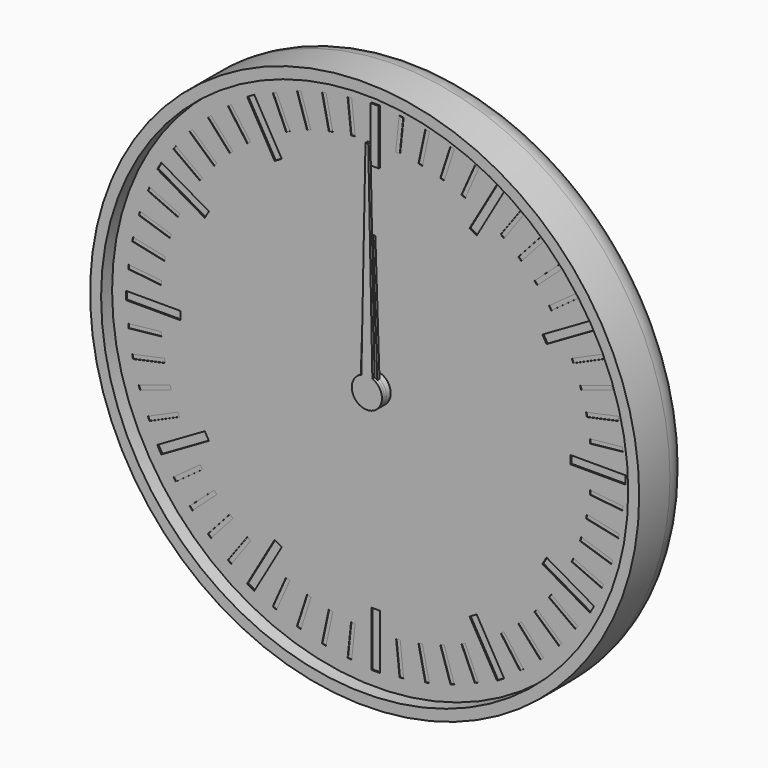
from build123d import *

# Parameters (mm, degrees)
F0_R      = 100
F1_DEPTH  = 24
F2_R      = 10
F3_T      = -4
F4_R      = 5.5
F4_R_2    = 3
F5_DEPTH  = 2
F6_DEPTH  = 19
F7_DEPTH  = 8
F9_DEPTH  = 4
F11_DEPTH = 4
F12_R     = 5.5
F12_R_2   = 3
F13_DEPTH = 2
F14_R     = 3
F15_DEPTH = 4
F17_DEPTH = 4
F18_R     = 3
F19_DEPTH = 2
F20_R     = 98
F20_R_2   = 5.5
F21_DEPTH = 1
F23_R     = 5
F23_R_2   = 3
F24_DEPTH = 2
F25_W     = 3
F25_H     = 20
F25_W_2   = 20
F25_H_2   = 3
F26_DEPTH = 0.5
F27_W     = 1.5
F27_H     = 12
F27_W_2   = 12
F27_H_2   = 1.5
F28_DEPTH = 0.2
F29_DEPTH = 1
F30_DEPTH = 0.4
F31_R     = 5.5
F31_R_2   = 3
F32_DEPTH = 5
F33_R     = 3
F34_DEPTH = 1
F36_DEPTH = 1


with BuildPart() as f1:
    # F0 (on Front) → F1 (new body)
    with BuildSketch(Plane.XZ):
        Circle(F0_R)
    extrude(amount=F1_DEPTH)

    # F2
    f2_edges = [f1.edges().sort_by_distance(p)[0] for p in [
        (-100, 0, 0),
    ]]
    fillet(f2_edges, radius=F2_R)

    # F3
    f3_openings = [f1.faces().sort_by_distance(p)[0] for p in [
        (0, -24, 0),
    ]]
    offset(amount=F3_T, openings=f3_openings)

    # F4 (on face) → F5 (join)
    with BuildSketch(Plane.XZ.offset(4)):
        Circle(F4_R)
        Circle(F4_R_2, mode=Mode.SUBTRACT)
        with Locations((40, 0)):
            Circle(F4_R)
        with Locations((40, 0)):
            Circle(F4_R_2, mode=Mode.SUBTRACT)
    extrude(amount=F5_DEPTH)


with BuildPart() as f6:
    # F6 (new): a face of the model
    f6_faces = [f1.part.faces().sort_by_distance(p)[0] for p in [
        (0, -4, 0),
    ]]
    extrude(f6_faces, amount=F6_DEPTH)

    # F8 (on face) → F9 (join)
    with BuildSketch(Plane.XZ.offset(6)):
        with BuildLine():
            ThreePointArc((9.2729637667, -1.3794085621), (9.3494561423, -0.6915886375), (9.375, 0))
            ThreePointArc((9.375, 0), (9.3494561423, 0.6915886375), (9.2729637667, 1.3794085621))
            ThreePointArc((9.2729637667, 1.3794085621), (8.9161548403, 2.8970343223), (8.3127812852, 4.3345463782))
            ThreePointArc((8.3127812852, 4.3345463782), (7.5845343223, 5.5104867402), (6.6911892658, 6.566476316))
            ThreePointArc((6.6911892658, 6.566476316), (5.5104867402, 7.5845343223), (4.1773988938, 8.3928519278))
            ThreePointArc((4.1773988938, 8.3928519278), (2.8970343223, 8.9161548403), (1.5536078905, 9.2453733036))
            ThreePointArc((1.5536078905, 9.2453733036), (0, 9.375), (-1.5536078905, 9.2453733036))
            ThreePointArc((-1.5536078905, 9.2453733036), (-2.8970343223, 8.9161548403), (-4.1773988938, 8.3928519278))
            ThreePointArc((-4.1773988938, 8.3928519278), (-5.5104867402, 7.5845343223), (-6.6911892658, 6.566476316))
            ThreePointArc((-6.6911892658, 6.566476316), (-7.5845343223, 5.5104867402), (-8.3127812852, 4.3345463782))
            ThreePointArc((-8.3127812852, 4.3345463782), (-8.9161548403, 2.8970343223), (-9.2729637667, 1.3794085621))
            ThreePointArc((-9.2729637667, 1.3794085621), (-9.375, 0), (-9.2729637667, -1.3794085621))
            ThreePointArc((-9.2729637667, -1.3794085621), (-8.9161548403, -2.8970343223), (-8.3127812852, -4.3345463782))
            ThreePointArc((-8.3127812852, -4.3345463782), (-7.5845343223, -5.5104867402), (-6.6911892658, -6.566476316))
            ThreePointArc((-6.6911892658, -6.566476316), (-5.5104867402, -7.5845343223), (-4.1773988938, -8.3928519278))
            ThreePointArc((-4.1773988938, -8.3928519278), (-2.8970343223, -8.9161548403), (-1.5536078905, -9.2453733036))
            ThreePointArc((-1.5536078905, -9.2453733036), (0, -9.375), (1.5536078905, -9.2453733036))
            ThreePointArc((1.5536078905, -9.2453733036), (2.8970343223, -8.9161548403), (4.1773988938, -8.3928519278))
            ThreePointArc((4.1773988938, -8.3928519278), (5.5104867402, -7.5845343223), (6.6911892658, -6.566476316))
            ThreePointArc((6.6911892658, -6.566476316), (7.5845343223, -5.5104867402), (8.3127812852, -4.3345463782))
            ThreePointArc((8.3127812852, -4.3345463782), (8.9161548403, -2.8970343223), (9.2729637667, -1.3794085621))
        make_face()
        with BuildLine():
            ThreePointArc((8.3127812852, 4.3345463782), (8.9161548403, 2.8970343223), (9.2729637667, 1.3794085621))
            Line((9.2729637667, 1.3794085621), (11.1823199426, 2.3946312492))
            Line((11.1823199426, 2.3946312492), (10.8182678729, 3.515068311))
            Line((10.8182678729, 3.515068311), (10.4542158031, 4.6355053728))
            Line((10.4542158031, 4.6355053728), (8.3127812852, 4.3345463782))
        make_face()
        with BuildLine():
            Line((11.1823199426, -2.3946312492), (9.2729637667, -1.3794085621))
            ThreePointArc((9.2729637667, -1.3794085621), (8.9161548403, -2.8970343223), (8.3127812852, -4.3345463782))
            Line((8.3127812852, -4.3345463782), (10.4542158031, -4.6355053728))
            Line((10.4542158031, -4.6355053728), (10.8182678729, -3.515068311))
            Line((10.8182678729, -3.515068311), (11.1823199426, -2.3946312492))
        make_face()
        with BuildLine():
            ThreePointArc((4.1773988938, 8.3928519278), (5.5104867402, 7.5845343223), (6.6911892658, 6.566476316))
            Line((6.6911892658, 6.566476316), (7.6391579371, 8.5101001246))
            Line((7.6391579371, 8.5101001246), (6.6860572448, 9.202568311))
            Line((6.6860572448, 9.202568311), (5.7329565525, 9.8950364974))
            Line((5.7329565525, 9.8950364974), (4.1773988938, 8.3928519278))
        make_face()
        with BuildLine():
            Line((7.6391579371, -8.5101001246), (6.6911892658, -6.566476316))
            ThreePointArc((6.6911892658, -6.566476316), (5.5104867402, -7.5845343223), (4.1773988938, -8.3928519278))
            Line((4.1773988938, -8.3928519278), (5.7329565525, -9.8950364974))
            Line((5.7329565525, -9.8950364974), (6.6860572448, -9.202568311))
            Line((6.6860572448, -9.202568311), (7.6391579371, -8.5101001246))
        make_face()
        with BuildLine():
            ThreePointArc((-1.5536078905, 9.2453733036), (0, 9.375), (1.5536078905, 9.2453733036))
            Line((1.5536078905, 9.2453733036), (1.1780972451, 11.375))
            Line((1.1780972451, 11.375), (0, 11.375))
            Line((0, 11.375), (-1.1780972451, 11.375))
            Line((-1.1780972451, 11.375), (-1.5536078905, 9.2453733036))
        make_face()
        with BuildLine():
            Line((1.1780972451, -11.375), (1.5536078905, -9.2453733036))
            ThreePointArc((1.5536078905, -9.2453733036), (0, -9.375), (-1.5536078905, -9.2453733036))
            Line((-1.5536078905, -9.2453733036), (-1.1780972451, -11.375))
            Line((-1.1780972451, -11.375), (0, -11.375))
            Line((0, -11.375), (1.1780972451, -11.375))
        make_face()
        with BuildLine():
            ThreePointArc((-6.6911892658, 6.566476316), (-5.5104867402, 7.5845343223), (-4.1773988938, 8.3928519278))
            Line((-4.1773988938, 8.3928519278), (-5.7329565525, 9.8950364974))
            Line((-5.7329565525, 9.8950364974), (-6.6860572448, 9.202568311))
            Line((-6.6860572448, 9.202568311), (-7.6391579371, 8.5101001246))
            Line((-7.6391579371, 8.5101001246), (-6.6911892658, 6.566476316))
        make_face()
        with BuildLine():
            Line((-5.7329565525, -9.8950364974), (-4.1773988938, -8.3928519278))
            ThreePointArc((-4.1773988938, -8.3928519278), (-5.5104867402, -7.5845343223), (-6.6911892658, -6.566476316))
            Line((-6.6911892658, -6.566476316), (-7.6391579371, -8.5101001246))
            Line((-7.6391579371, -8.5101001246), (-6.6860572448, -9.202568311))
            Line((-6.6860572448, -9.202568311), (-5.7329565525, -9.8950364974))
        make_face()
        with BuildLine():
            ThreePointArc((-9.2729637667, 1.3794085621), (-8.9161548403, 2.8970343223), (-8.3127812852, 4.3345463782))
            Line((-8.3127812852, 4.3345463782), (-10.4542158031, 4.6355053728))
            Line((-10.4542158031, 4.6355053728), (-10.8182678729, 3.515068311))
            Line((-10.8182678729, 3.515068311), (-11.1823199426, 2.3946312492))
            Line((-11.1823199426, 2.3946312492), (-9.2729637667, 1.3794085621))
        make_face()
        with BuildLine():
            Line((-10.4542158031, -4.6355053728), (-8.3127812852, -4.3345463782))
            ThreePointArc((-8.3127812852, -4.3345463782), (-8.9161548403, -2.8970343223), (-9.2729637667, -1.3794085621))
            Line((-9.2729637667, -1.3794085621), (-11.1823199426, -2.3946312492))
            Line((-11.1823199426, -2.3946312492), (-10.8182678729, -3.515068311))
            Line((-10.8182678729, -3.515068311), (-10.4542158031, -4.6355053728))
        make_face()
    extrude(amount=F9_DEPTH)

    # F35 (on face) → F36 (join)
    with BuildSketch(Plane.XZ.offset(23)):
        with BuildLine():
            ThreePointArc((-2, 5.123475383), (-3.1024184115, -4.5414755311), (5.5, 0))
            ThreePointArc((5.5, 0), (4.5414755311, 3.1024184115), (2, 5.123475383))
            ThreePointArc((2, 5.123475383), (0, 5.5), (-2, 5.123475383))
        make_face()
        with BuildLine():
            ThreePointArc((-2, 5.123475383), (0, 5.5), (2, 5.123475383))
            Line((2, 5.123475383), (0.5, 80))
            Line((0.5, 80), (0, 80))
            Line((0, 80), (-0.5, 80))
            Line((-0.5, 80), (-2, 5.123475383))
        make_face()
    extrude(amount=-F36_DEPTH)


with BuildPart() as f7:
    # F7 (new): a face of the model
    f7_faces = [f1.part.faces().sort_by_distance(p)[0] for p in [
        (40, -4, 0),
    ]]
    extrude(f7_faces, amount=F7_DEPTH)

    # F10 (on face) → F11 (join)
    with BuildSketch(Plane.XZ.offset(6)):
        with BuildLine():
            ThreePointArc((68.0829066802, -1.5381733945), (68.1144747006, -0.7693746225), (68.125, 0))
            ThreePointArc((68.125, 0), (68.1144747006, 0.7693746225), (68.0829066802, 1.5381733945))
            ThreePointArc((68.0829066802, 1.5381733945), (67.9709283072, 2.9398630294), (67.7890320221, 4.3342039956))
            ThreePointArc((67.7890320221, 4.3342039956), (67.5104012706, 5.8475163042), (67.1494235596, 7.3433252263))
            ThreePointArc((67.1494235596, 7.3433252263), (66.7484645208, 8.6911029668), (66.280643318, 10.0171558733))
            ThreePointArc((66.280643318, 10.0171558733), (65.6934659962, 11.4394680865), (65.0293803521, 12.8275385085))
            ThreePointArc((65.0293803521, 12.8275385085), (64.3569644814, 14.0625), (63.6236643925, 15.2623099717))
            ThreePointArc((63.6236643925, 15.2623099717), (62.7536029668, 16.5314602207), (61.815433119, 17.7511268046))
            ThreePointArc((61.815433119, 17.7511268046), (60.9009482166, 18.8192983038), (59.934217974, 19.8404278876))
            ThreePointArc((59.934217974, 19.8404278876), (58.8192983038, 20.9009482166), (57.6480467764, 21.8989056799))
            ThreePointArc((57.6480467764, 21.8989056799), (56.5314602207, 22.7536029668), (55.3735505752, 23.5514238999))
            ThreePointArc((55.3735505752, 23.5514238999), (54.0625, 24.3569644814), (52.709356105, 25.0895972944))
            ThreePointArc((52.709356105, 25.0895972944), (51.4394680865, 25.6934659962), (50.1409852457, 26.2331096755))
            ThreePointArc((50.1409852457, 26.2331096755), (48.6911029668, 26.7484645208), (47.2152055856, 27.1837531139))
            ThreePointArc((47.2152055856, 27.1837531139), (45.8475163042, 27.5104012706), (44.4652101991, 27.7682826779))
            ThreePointArc((44.4652101991, 27.7682826779), (42.9398630294, 27.9709283072), (41.4057159597, 28.0898484802))
            ThreePointArc((41.4057159597, 28.0898484802), (40, 28.125), (38.5942840403, 28.0898484802))
            ThreePointArc((38.5942840403, 28.0898484802), (37.0601369706, 27.9709283072), (35.5347898009, 27.7682826779))
            ThreePointArc((35.5347898009, 27.7682826779), (34.1524836958, 27.5104012706), (32.7847944144, 27.1837531139))
            ThreePointArc((32.7847944144, 27.1837531139), (31.3088970332, 26.7484645208), (29.8590147543, 26.2331096755))
            ThreePointArc((29.8590147543, 26.2331096755), (28.5605319135, 25.6934659962), (27.290643895, 25.0895972944))
            ThreePointArc((27.290643895, 25.0895972944), (25.9375, 24.3569644814), (24.6264494248, 23.5514238999))
            ThreePointArc((24.6264494248, 23.5514238999), (23.4685397793, 22.7536029668), (22.3519532236, 21.8989056799))
            ThreePointArc((22.3519532236, 21.8989056799), (21.1807016962, 20.9009482166), (20.065782026, 19.8404278876))
            ThreePointArc((20.065782026, 19.8404278876), (19.0990517834, 18.8192983038), (18.184566881, 17.7511268046))
            ThreePointArc((18.184566881, 17.7511268046), (17.2463970332, 16.5314602207), (16.3763356075, 15.2623099717))
            ThreePointArc((16.3763356075, 15.2623099717), (15.6430355186, 14.0625), (14.9706196479, 12.8275385085))
            ThreePointArc((14.9706196479, 12.8275385085), (14.3065340038, 11.4394680865), (13.719356682, 10.0171558733))
            ThreePointArc((13.719356682, 10.0171558733), (13.2515354792, 8.6911029668), (12.8505764404, 7.3433252263))
            ThreePointArc((12.8505764404, 7.3433252263), (12.4895987294, 5.8475163042), (12.2109679779, 4.3342039956))
            ThreePointArc((12.2109679779, 4.3342039956), (12.0290716928, 2.9398630294), (11.9170933198, 1.5381733945))
            ThreePointArc((11.9170933198, 1.5381733945), (11.875, 0), (11.9170933198, -1.5381733945))
            ThreePointArc((11.9170933198, -1.5381733945), (12.0290716928, -2.9398630294), (12.2109679779, -4.3342039956))
            ThreePointArc((12.2109679779, -4.3342039956), (12.4895987294, -5.8475163042), (12.8505764404, -7.3433252263))
            ThreePointArc((12.8505764404, -7.3433252263), (13.2515354792, -8.6911029668), (13.719356682, -10.0171558733))
            ThreePointArc((13.719356682, -10.0171558733), (14.3065340038, -11.4394680865), (14.9706196479, -12.8275385085))
            ThreePointArc((14.9706196479, -12.8275385085), (15.6430355186, -14.0625), (16.3763356075, -15.2623099717))
            ThreePointArc((16.3763356075, -15.2623099717), (17.2463970332, -16.5314602207), (18.184566881, -17.7511268046))
            ThreePointArc((18.184566881, -17.7511268046), (19.0990517834, -18.8192983038), (20.065782026, -19.8404278876))
            ThreePointArc((20.065782026, -19.8404278876), (21.1807016962, -20.9009482166), (22.3519532236, -21.8989056799))
            ThreePointArc((22.3519532236, -21.8989056799), (23.4685397793, -22.7536029668), (24.6264494248, -23.5514238999))
            ThreePointArc((24.6264494248, -23.5514238999), (25.9375, -24.3569644814), (27.290643895, -25.0895972944))
            ThreePointArc((27.290643895, -25.0895972944), (28.5605319135, -25.6934659962), (29.8590147543, -26.2331096755))
            ThreePointArc((29.8590147543, -26.2331096755), (31.3088970332, -26.7484645208), (32.7847944144, -27.1837531139))
            ThreePointArc((32.7847944144, -27.1837531139), (34.1524836958, -27.5104012706), (35.5347898009, -27.7682826779))
            ThreePointArc((35.5347898009, -27.7682826779), (37.0601369706, -27.9709283072), (38.5942840403, -28.0898484802))
            ThreePointArc((38.5942840403, -28.0898484802), (40, -28.125), (41.4057159597, -28.0898484802))
            ThreePointArc((41.4057159597, -28.0898484802), (42.9398630294, -27.9709283072), (44.4652101991, -27.7682826779))
            ThreePointArc((44.4652101991, -27.7682826779), (45.8475163042, -27.5104012706), (47.2152055856, -27.1837531139))
            ThreePointArc((47.2152055856, -27.1837531139), (48.6911029668, -26.7484645208), (50.1409852457, -26.2331096755))
            ThreePointArc((50.1409852457, -26.2331096755), (51.4394680865, -25.6934659962), (52.709356105, -25.0895972944))
            ThreePointArc((52.709356105, -25.0895972944), (54.0625, -24.3569644814), (55.3735505752, -23.5514238999))
            ThreePointArc((55.3735505752, -23.5514238999), (56.5314602207, -22.7536029668), (57.6480467764, -21.8989056799))
            ThreePointArc((57.6480467764, -21.8989056799), (58.8192983038, -20.9009482166), (59.934217974, -19.8404278876))
            ThreePointArc((59.934217974, -19.8404278876), (60.9009482166, -18.8192983038), (61.815433119, -17.7511268046))
            ThreePointArc((61.815433119, -17.7511268046), (62.7536029668, -16.5314602207), (63.6236643925, -15.2623099717))
            ThreePointArc((63.6236643925, -15.2623099717), (64.3569644814, -14.0625), (65.0293803521, -12.8275385085))
            ThreePointArc((65.0293803521, -12.8275385085), (65.6934659962, -11.4394680865), (66.280643318, -10.0171558733))
            ThreePointArc((66.280643318, -10.0171558733), (66.7484645208, -8.6911029668), (67.1494235596, -7.3433252263))
            ThreePointArc((67.1494235596, -7.3433252263), (67.5104012706, -5.8475163042), (67.7890320221, -4.3342039956))
            ThreePointArc((67.7890320221, -4.3342039956), (67.9709283072, -2.9398630294), (68.0829066802, -1.5381733945))
        make_face()
        with BuildLine():
            ThreePointArc((68.0829066802, 1.5381733945), (68.1144747006, 0.7693746225), (68.125, 0))
            ThreePointArc((68.125, 0), (68.1144747006, -0.7693746225), (68.0829066802, -1.5381733945))
            Line((68.0829066802, -1.5381733945), (70.125, -1.1780972451))
            Line((70.125, -1.1780972451), (70.125, 0))
            Line((70.125, 0), (70.125, 1.1780972451))
            Line((70.125, 1.1780972451), (68.0829066802, 1.5381733945))
        make_face()
        with BuildLine():
            ThreePointArc((67.1494235596, 7.3433252263), (67.5104012706, 5.8475163042), (67.7890320221, 4.3342039956))
            Line((67.7890320221, 4.3342039956), (69.7116366623, 5.1109866922))
            Line((69.7116366623, 5.1109866922), (69.4666964721, 6.2633396859))
            Line((69.4666964721, 6.2633396859), (69.2217562819, 7.4156926796))
            Line((69.2217562819, 7.4156926796), (67.1494235596, 7.3433252263))
        make_face()
        with BuildLine():
            Line((69.7116366623, -5.1109866922), (67.7890320221, -4.3342039956))
            ThreePointArc((67.7890320221, -4.3342039956), (67.5104012706, -5.8475163042), (67.1494235596, -7.3433252263))
            Line((67.1494235596, -7.3433252263), (69.2217562819, -7.4156926796))
            Line((69.2217562819, -7.4156926796), (69.4666964721, -6.2633396859))
            Line((69.4666964721, -6.2633396859), (69.7116366623, -5.1109866922))
        make_face()
        with BuildLine():
            ThreePointArc((65.0293803521, 12.8275385085), (65.6934659962, 11.4394680865), (66.280643318, 10.0171558733))
            Line((66.280643318, 10.0171558733), (67.9997322302, 11.1766959857))
            Line((67.9997322302, 11.1766959857), (67.5205569115, 12.2529413727))
            Line((67.5205569115, 12.2529413727), (67.0413815928, 13.3291867596))
            Line((67.0413815928, 13.3291867596), (65.0293803521, 12.8275385085))
        make_face()
        with BuildLine():
            Line((67.9997322302, -11.1766959857), (66.280643318, -10.0171558733))
            ThreePointArc((66.280643318, -10.0171558733), (65.6934659962, -11.4394680865), (65.0293803521, -12.8275385085))
            Line((65.0293803521, -12.8275385085), (67.0413815928, -13.3291867596))
            Line((67.0413815928, -13.3291867596), (67.5205569115, -12.2529413727))
            Line((67.5205569115, -12.2529413727), (67.9997322302, -11.1766959857))
        make_face()
        with BuildLine():
            ThreePointArc((61.815433119, 17.7511268046), (62.7536029668, 16.5314602207), (63.6236643925, 15.2623099717))
            Line((63.6236643925, 15.2623099717), (65.064105142, 16.753930033))
            Line((65.064105142, 16.753930033), (64.3716369555, 17.7070307253))
            Line((64.3716369555, 17.7070307253), (63.6791687691, 18.6601314176))
            Line((63.6791687691, 18.6601314176), (61.815433119, 17.7511268046))
        make_face()
        with BuildLine():
            Line((65.064105142, -16.753930033), (63.6236643925, -15.2623099717))
            ThreePointArc((63.6236643925, -15.2623099717), (62.7536029668, -16.5314602207), (61.815433119, -17.7511268046))
            Line((61.815433119, -17.7511268046), (63.6791687691, -18.6601314176))
            Line((63.6791687691, -18.6601314176), (64.3716369555, -17.7070307253))
            Line((64.3716369555, -17.7070307253), (65.064105142, -16.753930033))
        make_face()
        with BuildLine():
            ThreePointArc((57.6480467764, 21.8989056799), (58.8192983038, 20.9009482166), (59.934217974, 19.8404278876))
            Line((59.934217974, 19.8404278876), (61.0330563882, 21.5989369435))
            Line((61.0330563882, 21.5989369435), (60.1575595166, 22.3872378675))
            Line((60.1575595166, 22.3872378675), (59.282062645, 23.1755387915))
            Line((59.282062645, 23.1755387915), (57.6480467764, 21.8989056799))
        make_face()
        with BuildLine():
            Line((61.0330563882, -21.5989369435), (59.934217974, -19.8404278876))
            ThreePointArc((59.934217974, -19.8404278876), (58.8192983038, -20.9009482166), (57.6480467764, -21.8989056799))
            Line((57.6480467764, -21.8989056799), (59.282062645, -23.1755387915))
            Line((59.282062645, -23.1755387915), (60.1575595166, -22.3872378675))
            Line((60.1575595166, -22.3872378675), (61.0330563882, -21.5989369435))
        make_face()
        with BuildLine():
            ThreePointArc((52.709356105, 25.0895972944), (54.0625, 24.3569644814), (55.3735505752, 23.5514238999))
            Line((55.3735505752, 23.5514238999), (56.0827621424, 25.4999666665))
            Line((56.0827621424, 25.4999666665), (55.0625, 26.089015289))
            Line((55.0625, 26.089015289), (54.0422378576, 26.6780639116))
            Line((54.0422378576, 26.6780639116), (52.709356105, 25.0895972944))
        make_face()
        with BuildLine():
            Line((56.0827621424, -25.4999666665), (55.3735505752, -23.5514238999))
            ThreePointArc((55.3735505752, -23.5514238999), (54.0625, -24.3569644814), (52.709356105, -25.0895972944))
            Line((52.709356105, -25.0895972944), (54.0422378576, -26.6780639116))
            Line((54.0422378576, -26.6780639116), (55.0625, -26.089015289))
            Line((55.0625, -26.089015289), (56.0827621424, -25.4999666665))
        make_face()
        with BuildLine():
            ThreePointArc((47.2152055856, 27.1837531139), (48.6911029668, 26.7484645208), (50.1409852457, 26.2331096755))
            Line((50.1409852457, 26.2331096755), (50.4295740173, 28.2865254836))
            Line((50.4295740173, 28.2865254836), (49.3091369555, 28.6505775534))
            Line((49.3091369555, 28.6505775534), (48.1886998938, 29.0146296232))
            Line((48.1886998938, 29.0146296232), (47.2152055856, 27.1837531139))
        make_face()
        with BuildLine():
            Line((50.4295740173, -28.2865254836), (50.1409852457, -26.2331096755))
            ThreePointArc((50.1409852457, -26.2331096755), (48.6911029668, -26.7484645208), (47.2152055856, -27.1837531139))
            Line((47.2152055856, -27.1837531139), (48.1886998938, -29.0146296232))
            Line((48.1886998938, -29.0146296232), (49.3091369555, -28.6505775534))
            Line((49.3091369555, -28.6505775534), (50.4295740173, -28.2865254836))
        make_face()
        with BuildLine():
            ThreePointArc((41.4057159597, 28.0898484802), (42.9398630294, 27.9709283072), (44.4652101991, 27.7682826779))
            Line((44.4652101991, 27.7682826779), (44.3205634611, 29.8368274034))
            Line((44.3205634611, 29.8368274034), (43.1489199559, 29.959972098))
            Line((43.1489199559, 29.959972098), (41.9772764508, 30.0831167926))
            Line((41.9772764508, 30.0831167926), (41.4057159597, 28.0898484802))
        make_face()
        with BuildLine():
            Line((44.3205634611, -29.8368274034), (44.4652101991, -27.7682826779))
            ThreePointArc((44.4652101991, -27.7682826779), (42.9398630294, -27.9709283072), (41.4057159597, -28.0898484802))
            Line((41.4057159597, -28.0898484802), (41.9772764508, -30.0831167926))
            Line((41.9772764508, -30.0831167926), (43.1489199559, -29.959972098))
            Line((43.1489199559, -29.959972098), (44.3205634611, -29.8368274034))
        make_face()
        with BuildLine():
            ThreePointArc((35.5347898009, 27.7682826779), (37.0601369706, 27.9709283072), (38.5942840403, 28.0898484802))
            Line((38.5942840403, 28.0898484802), (38.0227235492, 30.0831167926))
            Line((38.0227235492, 30.0831167926), (36.8510800441, 29.959972098))
            Line((36.8510800441, 29.959972098), (35.6794365389, 29.8368274034))
            Line((35.6794365389, 29.8368274034), (35.5347898009, 27.7682826779))
        make_face()
        with BuildLine():
            Line((38.0227235492, -30.0831167926), (38.5942840403, -28.0898484802))
            ThreePointArc((38.5942840403, -28.0898484802), (37.0601369706, -27.9709283072), (35.5347898009, -27.7682826779))
            Line((35.5347898009, -27.7682826779), (35.6794365389, -29.8368274034))
            Line((35.6794365389, -29.8368274034), (36.8510800441, -29.959972098))
            Line((36.8510800441, -29.959972098), (38.0227235492, -30.0831167926))
        make_face()
        with BuildLine():
            ThreePointArc((29.8590147543, 26.2331096755), (31.3088970332, 26.7484645208), (32.7847944144, 27.1837531139))
            Line((32.7847944144, 27.1837531139), (31.8113001062, 29.0146296232))
            Line((31.8113001062, 29.0146296232), (30.6908630445, 28.6505775534))
            Line((30.6908630445, 28.6505775534), (29.5704259827, 28.2865254836))
            Line((29.5704259827, 28.2865254836), (29.8590147543, 26.2331096755))
        make_face()
        with BuildLine():
            Line((31.8113001062, -29.0146296232), (32.7847944144, -27.1837531139))
            ThreePointArc((32.7847944144, -27.1837531139), (31.3088970332, -26.7484645208), (29.8590147543, -26.2331096755))
            Line((29.8590147543, -26.2331096755), (29.5704259827, -28.2865254836))
            Line((29.5704259827, -28.2865254836), (30.6908630445, -28.6505775534))
            Line((30.6908630445, -28.6505775534), (31.8113001062, -29.0146296232))
        make_face()
        with BuildLine():
            ThreePointArc((24.6264494248, 23.5514238999), (25.9375, 24.3569644814), (27.290643895, 25.0895972944))
            Line((27.290643895, 25.0895972944), (25.9577621424, 26.6780639116))
            Line((25.9577621424, 26.6780639116), (24.9375, 26.089015289))
            Line((24.9375, 26.089015289), (23.9172378576, 25.4999666665))
            Line((23.9172378576, 25.4999666665), (24.6264494248, 23.5514238999))
        make_face()
        with BuildLine():
            Line((25.9577621424, -26.6780639116), (27.290643895, -25.0895972944))
            ThreePointArc((27.290643895, -25.0895972944), (25.9375, -24.3569644814), (24.6264494248, -23.5514238999))
            Line((24.6264494248, -23.5514238999), (23.9172378576, -25.4999666665))
            Line((23.9172378576, -25.4999666665), (24.9375, -26.089015289))
            Line((24.9375, -26.089015289), (25.9577621424, -26.6780639116))
        make_face()
        with BuildLine():
            ThreePointArc((20.065782026, 19.8404278876), (21.1807016962, 20.9009482166), (22.3519532236, 21.8989056799))
            Line((22.3519532236, 21.8989056799), (20.717937355, 23.1755387915))
            Line((20.717937355, 23.1755387915), (19.8424404834, 22.3872378675))
            Line((19.8424404834, 22.3872378675), (18.9669436118, 21.5989369435))
            Line((18.9669436118, 21.5989369435), (20.065782026, 19.8404278876))
        make_face()
        with BuildLine():
            Line((20.717937355, -23.1755387915), (22.3519532236, -21.8989056799))
            ThreePointArc((22.3519532236, -21.8989056799), (21.1807016962, -20.9009482166), (20.065782026, -19.8404278876))
            Line((20.065782026, -19.8404278876), (18.9669436118, -21.5989369435))
            Line((18.9669436118, -21.5989369435), (19.8424404834, -22.3872378675))
            Line((19.8424404834, -22.3872378675), (20.717937355, -23.1755387915))
        make_face()
        with BuildLine():
            ThreePointArc((16.3763356075, 15.2623099717), (17.2463970332, 16.5314602207), (18.184566881, 17.7511268046))
            Line((18.184566881, 17.7511268046), (16.3208312309, 18.6601314176))
            Line((16.3208312309, 18.6601314176), (15.6283630445, 17.7070307253))
            Line((15.6283630445, 17.7070307253), (14.935894858, 16.753930033))
            Line((14.935894858, 16.753930033), (16.3763356075, 15.2623099717))
        make_face()
        with BuildLine():
            Line((16.3208312309, -18.6601314176), (18.184566881, -17.7511268046))
            ThreePointArc((18.184566881, -17.7511268046), (17.2463970332, -16.5314602207), (16.3763356075, -15.2623099717))
            Line((16.3763356075, -15.2623099717), (14.935894858, -16.753930033))
            Line((14.935894858, -16.753930033), (15.6283630445, -17.7070307253))
            Line((15.6283630445, -17.7070307253), (16.3208312309, -18.6601314176))
        make_face()
        with BuildLine():
            ThreePointArc((13.719356682, 10.0171558733), (14.3065340038, 11.4394680865), (14.9706196479, 12.8275385085))
            Line((14.9706196479, 12.8275385085), (12.9586184072, 13.3291867596))
            Line((12.9586184072, 13.3291867596), (12.4794430885, 12.2529413727))
            Line((12.4794430885, 12.2529413727), (12.0002677698, 11.1766959857))
            Line((12.0002677698, 11.1766959857), (13.719356682, 10.0171558733))
        make_face()
        with BuildLine():
            Line((12.9586184072, -13.3291867596), (14.9706196479, -12.8275385085))
            ThreePointArc((14.9706196479, -12.8275385085), (14.3065340038, -11.4394680865), (13.719356682, -10.0171558733))
            Line((13.719356682, -10.0171558733), (12.0002677698, -11.1766959857))
            Line((12.0002677698, -11.1766959857), (12.4794430885, -12.2529413727))
            Line((12.4794430885, -12.2529413727), (12.9586184072, -13.3291867596))
        make_face()
        with BuildLine():
            ThreePointArc((12.2109679779, 4.3342039956), (12.4895987294, 5.8475163042), (12.8505764404, 7.3433252263))
            Line((12.8505764404, 7.3433252263), (10.7782437181, 7.4156926796))
            Line((10.7782437181, 7.4156926796), (10.5333035279, 6.2633396859))
            Line((10.5333035279, 6.2633396859), (10.2883633377, 5.1109866922))
            Line((10.2883633377, 5.1109866922), (12.2109679779, 4.3342039956))
        make_face()
        with BuildLine():
            Line((10.7782437181, -7.4156926796), (12.8505764404, -7.3433252263))
            ThreePointArc((12.8505764404, -7.3433252263), (12.4895987294, -5.8475163042), (12.2109679779, -4.3342039956))
            Line((12.2109679779, -4.3342039956), (10.2883633377, -5.1109866922))
            Line((10.2883633377, -5.1109866922), (10.5333035279, -6.2633396859))
            Line((10.5333035279, -6.2633396859), (10.7782437181, -7.4156926796))
        make_face()
        with BuildLine():
            ThreePointArc((11.9170933198, -1.5381733945), (11.875, 0), (11.9170933198, 1.5381733945))
            Line((11.9170933198, 1.5381733945), (9.875, 1.1780972451))
            Line((9.875, 1.1780972451), (9.875, 0))
            Line((9.875, 0), (9.875, -1.1780972451))
            Line((9.875, -1.1780972451), (11.9170933198, -1.5381733945))
        make_face()
    extrude(amount=F11_DEPTH)

    # F16 (on face) → F17 (join)
    with BuildSketch(Plane.XZ.offset(12)):
        with BuildLine():
            ThreePointArc((47.4288750323, -1.0304444454), (47.4821976298, -0.5164480894), (47.5, 0))
            ThreePointArc((47.5, 0), (47.4821976298, 0.5164480894), (47.4288750323, 1.0304444454))
            ThreePointArc((47.4288750323, 1.0304444454), (47.1329238722, 2.3176274578), (46.6157661985, 3.532936117))
            ThreePointArc((46.6157661985, 3.532936117), (46.0676274578, 4.4083893922), (45.4044061018, 5.2002302532))
            ThreePointArc((45.4044061018, 5.2002302532), (44.4083893922, 6.0676274578), (43.2756595386, 6.7468551628))
            ThreePointArc((43.2756595386, 6.7468551628), (42.3176274578, 7.1329238722), (41.3156377295, 7.3837048536))
            ThreePointArc((41.3156377295, 7.3837048536), (40, 7.5), (38.6843622705, 7.3837048536))
            ThreePointArc((38.6843622705, 7.3837048536), (37.6823725422, 7.1329238722), (36.7243404614, 6.7468551628))
            ThreePointArc((36.7243404614, 6.7468551628), (35.5916106078, 6.0676274578), (34.5955938982, 5.2002302532))
            ThreePointArc((34.5955938982, 5.2002302532), (33.9323725422, 4.4083893922), (33.3842338015, 3.532936117))
            ThreePointArc((33.3842338015, 3.532936117), (32.8670761278, 2.3176274578), (32.5711249677, 1.0304444454))
            ThreePointArc((32.5711249677, 1.0304444454), (32.5, 0), (32.5711249677, -1.0304444454))
            ThreePointArc((32.5711249677, -1.0304444454), (32.8670761278, -2.3176274578), (33.3842338015, -3.532936117))
            ThreePointArc((33.3842338015, -3.532936117), (33.9323725422, -4.4083893922), (34.5955938982, -5.2002302532))
            ThreePointArc((34.5955938982, -5.2002302532), (35.5916106078, -6.0676274578), (36.7243404614, -6.7468551628))
            ThreePointArc((36.7243404614, -6.7468551628), (37.6823725422, -7.1329238722), (38.6843622705, -7.3837048536))
            ThreePointArc((38.6843622705, -7.3837048536), (40, -7.5), (41.3156377295, -7.3837048536))
            ThreePointArc((41.3156377295, -7.3837048536), (42.3176274578, -7.1329238722), (43.2756595386, -6.7468551628))
            ThreePointArc((43.2756595386, -6.7468551628), (44.4083893922, -6.0676274578), (45.4044061018, -5.2002302532))
            ThreePointArc((45.4044061018, -5.2002302532), (46.0676274578, -4.4083893922), (46.6157661985, -3.532936117))
            ThreePointArc((46.6157661985, -3.532936117), (47.1329238722, -2.3176274578), (47.4288750323, -1.0304444454))
        make_face()
        with BuildLine():
            ThreePointArc((46.6157661985, 3.532936117), (47.1329238722, 2.3176274578), (47.4288750323, 1.0304444454))
            Line((47.4288750323, 1.0304444454), (49.3262785606, 2.0393117971))
            Line((49.3262785606, 2.0393117971), (48.743795249, 3.832011096))
            Line((48.743795249, 3.832011096), (46.6157661985, 3.532936117))
        make_face()
        with BuildLine():
            Line((49.3262785606, -2.0393117971), (47.4288750323, -1.0304444454))
            ThreePointArc((47.4288750323, -1.0304444454), (47.1329238722, -2.3176274578), (46.6157661985, -3.532936117))
            Line((46.6157661985, -3.532936117), (48.743795249, -3.832011096))
            Line((48.743795249, -3.832011096), (49.3262785606, -2.0393117971))
        make_face()
        with BuildLine():
            ThreePointArc((43.2756595386, 6.7468551628), (44.4083893922, 6.0676274578), (45.4044061018, 5.2002302532))
            Line((45.4044061018, 5.2002302532), (46.3464404506, 7.1316868974))
            Line((46.3464404506, 7.1316868974), (44.8214793429, 8.2396359957))
            Line((44.8214793429, 8.2396359957), (43.2756595386, 6.7468551628))
        make_face()
        with BuildLine():
            Line((46.3464404506, -7.1316868974), (45.4044061018, -5.2002302532))
            ThreePointArc((45.4044061018, -5.2002302532), (44.4083893922, -6.0676274578), (43.2756595386, -6.7468551628))
            Line((43.2756595386, -6.7468551628), (44.8214793429, -8.2396359957))
            Line((44.8214793429, -8.2396359957), (46.3464404506, -7.1316868974))
        make_face()
        with BuildLine():
            ThreePointArc((38.6843622705, 7.3837048536), (40, 7.5), (41.3156377295, 7.3837048536))
            Line((41.3156377295, 7.3837048536), (40.9424777961, 9.5))
            Line((40.9424777961, 9.5), (39.0575222039, 9.5))
            Line((39.0575222039, 9.5), (38.6843622705, 7.3837048536))
        make_face()
        with BuildLine():
            Line((40.9424777961, -9.5), (41.3156377295, -7.3837048536))
            ThreePointArc((41.3156377295, -7.3837048536), (40, -7.5), (38.6843622705, -7.3837048536))
            Line((38.6843622705, -7.3837048536), (39.0575222039, -9.5))
            Line((39.0575222039, -9.5), (40.9424777961, -9.5))
        make_face()
        with BuildLine():
            ThreePointArc((34.5955938982, 5.2002302532), (35.5916106078, 6.0676274578), (36.7243404614, 6.7468551628))
            Line((36.7243404614, 6.7468551628), (35.1785206571, 8.2396359957))
            Line((35.1785206571, 8.2396359957), (33.6535595494, 7.1316868974))
            Line((33.6535595494, 7.1316868974), (34.5955938982, 5.2002302532))
        make_face()
        with BuildLine():
            Line((35.1785206571, -8.2396359957), (36.7243404614, -6.7468551628))
            ThreePointArc((36.7243404614, -6.7468551628), (35.5916106078, -6.0676274578), (34.5955938982, -5.2002302532))
            Line((34.5955938982, -5.2002302532), (33.6535595494, -7.1316868974))
            Line((33.6535595494, -7.1316868974), (35.1785206571, -8.2396359957))
        make_face()
        with BuildLine():
            ThreePointArc((32.5711249677, 1.0304444454), (32.8670761278, 2.3176274578), (33.3842338015, 3.532936117))
            Line((33.3842338015, 3.532936117), (31.256204751, 3.832011096))
            Line((31.256204751, 3.832011096), (30.6737214394, 2.0393117971))
            Line((30.6737214394, 2.0393117971), (32.5711249677, 1.0304444454))
        make_face()
        with BuildLine():
            Line((31.256204751, -3.832011096), (33.3842338015, -3.532936117))
            ThreePointArc((33.3842338015, -3.532936117), (32.8670761278, -2.3176274578), (32.5711249677, -1.0304444454))
            Line((32.5711249677, -1.0304444454), (30.6737214394, -2.0393117971))
            Line((30.6737214394, -2.0393117971), (31.256204751, -3.832011096))
        make_face()
    extrude(amount=F17_DEPTH)

    # F18 (on face) → F19 (join)
    with BuildSketch(Plane.XZ.offset(16)):
        with Locations((40, 0)):
            Circle(F18_R)
    extrude(amount=F19_DEPTH)


with BuildPart() as f13:
    # F12 (on face) → F13 (new body)
    with BuildSketch(Plane.XZ.offset(10)):
        Circle(F12_R)
        Circle(F12_R_2, mode=Mode.SUBTRACT)
    extrude(amount=F13_DEPTH)

    # F14 (on face) → F15 (join)
    with BuildSketch(Plane.XZ.offset(12)):
        with BuildLine():
            ThreePointArc((29.9718156995, -1.3001014101), (29.9929530972, -0.6502034357), (30, 0))
            ThreePointArc((30, 0), (29.9929530972, 0.6502034357), (29.9718156995, 1.3001014101))
            ThreePointArc((29.9718156995, 1.3001014101), (29.907520012, 2.3537728718), (29.8061935814, 3.4045299509))
            ThreePointArc((29.8061935814, 3.4045299509), (29.6306502179, 4.6930339512), (29.3994322443, 5.9727199596))
            ThreePointArc((29.3994322443, 5.9727199596), (29.1710976119, 7.0033609157), (28.9066440563, 8.0253304855))
            ThreePointArc((28.9066440563, 8.0253304855), (28.5316954889, 9.2705098312), (28.1031371961, 10.4982703213))
            ThreePointArc((28.1031371961, 10.4982703213), (27.7163859753, 11.480502971), (27.2953170189, 12.448520749))
            ThreePointArc((27.2953170189, 12.448520749), (26.7301957257, 13.6197149922), (26.1148496411, 14.765318426))
            ThreePointArc((26.1148496411, 14.765318426), (25.5792049306, 15.6749569415), (25.0118886885, 16.5651871174))
            ThreePointArc((25.0118886885, 16.5651871174), (24.2705098312, 17.6335575688), (23.4835278178, 18.6687953878))
            ThreePointArc((23.4835278178, 18.6687953878), (22.812178968, 19.4834414499), (22.1125846489, 20.2739636023))
            ThreePointArc((22.1125846489, 20.2739636023), (21.2132034356, 21.2132034356), (20.2739636023, 22.1125846489))
            ThreePointArc((20.2739636023, 22.1125846489), (19.4834414499, 22.812178968), (18.6687953878, 23.4835278178))
            ThreePointArc((18.6687953878, 23.4835278178), (17.6335575688, 24.2705098312), (16.5651871174, 25.0118886885))
            ThreePointArc((16.5651871174, 25.0118886885), (15.6749569415, 25.5792049306), (14.765318426, 26.1148496411))
            ThreePointArc((14.765318426, 26.1148496411), (13.6197149922, 26.7301957257), (12.448520749, 27.2953170189))
            ThreePointArc((12.448520749, 27.2953170189), (11.480502971, 27.7163859753), (10.4982703213, 28.1031371961))
            ThreePointArc((10.4982703213, 28.1031371961), (9.2705098312, 28.5316954889), (8.0253304855, 28.9066440563))
            ThreePointArc((8.0253304855, 28.9066440563), (7.0033609157, 29.1710976119), (5.9727199596, 29.3994322443))
            ThreePointArc((5.9727199596, 29.3994322443), (4.6930339512, 29.6306502179), (3.4045299509, 29.8061935814))
            ThreePointArc((3.4045299509, 29.8061935814), (2.3537728718, 29.907520012), (1.3001014101, 29.9718156995))
            ThreePointArc((1.3001014101, 29.9718156995), (0, 30), (-1.3001014101, 29.9718156995))
            ThreePointArc((-1.3001014101, 29.9718156995), (-2.3537728718, 29.907520012), (-3.4045299509, 29.8061935814))
            ThreePointArc((-3.4045299509, 29.8061935814), (-4.6930339512, 29.6306502179), (-5.9727199596, 29.3994322443))
            ThreePointArc((-5.9727199596, 29.3994322443), (-7.0033609157, 29.1710976119), (-8.0253304855, 28.9066440563))
            ThreePointArc((-8.0253304855, 28.9066440563), (-9.2705098312, 28.5316954889), (-10.4982703213, 28.1031371961))
            ThreePointArc((-10.4982703213, 28.1031371961), (-11.480502971, 27.7163859753), (-12.448520749, 27.2953170189))
            ThreePointArc((-12.448520749, 27.2953170189), (-13.6197149922, 26.7301957257), (-14.765318426, 26.1148496411))
            ThreePointArc((-14.765318426, 26.1148496411), (-15.6749569415, 25.5792049306), (-16.5651871174, 25.0118886885))
            ThreePointArc((-16.5651871174, 25.0118886885), (-17.6335575688, 24.2705098312), (-18.6687953878, 23.4835278178))
            ThreePointArc((-18.6687953878, 23.4835278178), (-19.4834414499, 22.812178968), (-20.2739636023, 22.1125846489))
            ThreePointArc((-20.2739636023, 22.1125846489), (-21.2132034356, 21.2132034356), (-22.1125846489, 20.2739636023))
            ThreePointArc((-22.1125846489, 20.2739636023), (-22.812178968, 19.4834414499), (-23.4835278178, 18.6687953878))
            ThreePointArc((-23.4835278178, 18.6687953878), (-24.2705098312, 17.6335575688), (-25.0118886885, 16.5651871174))
            ThreePointArc((-25.0118886885, 16.5651871174), (-25.5792049306, 15.6749569415), (-26.1148496411, 14.765318426))
            ThreePointArc((-26.1148496411, 14.765318426), (-26.7301957257, 13.6197149922), (-27.2953170189, 12.448520749))
            ThreePointArc((-27.2953170189, 12.448520749), (-27.7163859753, 11.480502971), (-28.1031371961, 10.4982703213))
            ThreePointArc((-28.1031371961, 10.4982703213), (-28.5316954889, 9.2705098312), (-28.9066440563, 8.0253304855))
            ThreePointArc((-28.9066440563, 8.0253304855), (-29.1710976119, 7.0033609157), (-29.3994322443, 5.9727199596))
            ThreePointArc((-29.3994322443, 5.9727199596), (-29.6306502179, 4.6930339512), (-29.8061935814, 3.4045299509))
            ThreePointArc((-29.8061935814, 3.4045299509), (-29.907520012, 2.3537728718), (-29.9718156995, 1.3001014101))
            ThreePointArc((-29.9718156995, 1.3001014101), (-30, 0), (-29.9718156995, -1.3001014101))
            ThreePointArc((-29.9718156995, -1.3001014101), (-29.907520012, -2.3537728718), (-29.8061935814, -3.4045299509))
            ThreePointArc((-29.8061935814, -3.4045299509), (-29.6306502179, -4.6930339512), (-29.3994322443, -5.9727199596))
            ThreePointArc((-29.3994322443, -5.9727199596), (-29.1710976119, -7.0033609157), (-28.9066440563, -8.0253304855))
            ThreePointArc((-28.9066440563, -8.0253304855), (-28.5316954889, -9.2705098312), (-28.1031371961, -10.4982703213))
            ThreePointArc((-28.1031371961, -10.4982703213), (-27.7163859753, -11.480502971), (-27.2953170189, -12.448520749))
            ThreePointArc((-27.2953170189, -12.448520749), (-26.7301957257, -13.6197149922), (-26.1148496411, -14.765318426))
            ThreePointArc((-26.1148496411, -14.765318426), (-25.5792049306, -15.6749569415), (-25.0118886885, -16.5651871174))
            ThreePointArc((-25.0118886885, -16.5651871174), (-24.2705098312, -17.6335575688), (-23.4835278178, -18.6687953878))
            ThreePointArc((-23.4835278178, -18.6687953878), (-22.812178968, -19.4834414499), (-22.1125846489, -20.2739636023))
            ThreePointArc((-22.1125846489, -20.2739636023), (-21.2132034356, -21.2132034356), (-20.2739636023, -22.1125846489))
            ThreePointArc((-20.2739636023, -22.1125846489), (-19.4834414499, -22.812178968), (-18.6687953878, -23.4835278178))
            ThreePointArc((-18.6687953878, -23.4835278178), (-17.6335575688, -24.2705098312), (-16.5651871174, -25.0118886885))
            ThreePointArc((-16.5651871174, -25.0118886885), (-15.6749569415, -25.5792049306), (-14.765318426, -26.1148496411))
            ThreePointArc((-14.765318426, -26.1148496411), (-13.6197149922, -26.7301957257), (-12.448520749, -27.2953170189))
            ThreePointArc((-12.448520749, -27.2953170189), (-11.480502971, -27.7163859753), (-10.4982703213, -28.1031371961))
            ThreePointArc((-10.4982703213, -28.1031371961), (-9.2705098312, -28.5316954889), (-8.0253304855, -28.9066440563))
            ThreePointArc((-8.0253304855, -28.9066440563), (-7.0033609157, -29.1710976119), (-5.9727199596, -29.3994322443))
            ThreePointArc((-5.9727199596, -29.3994322443), (-4.6930339512, -29.6306502179), (-3.4045299509, -29.8061935814))
            ThreePointArc((-3.4045299509, -29.8061935814), (-2.3537728718, -29.907520012), (-1.3001014101, -29.9718156995))
            ThreePointArc((-1.3001014101, -29.9718156995), (0, -30), (1.3001014101, -29.9718156995))
            ThreePointArc((1.3001014101, -29.9718156995), (2.3537728718, -29.907520012), (3.4045299509, -29.8061935814))
            ThreePointArc((3.4045299509, -29.8061935814), (4.6930339512, -29.6306502179), (5.9727199596, -29.3994322443))
            ThreePointArc((5.9727199596, -29.3994322443), (7.0033609157, -29.1710976119), (8.0253304855, -28.9066440563))
            ThreePointArc((8.0253304855, -28.9066440563), (9.2705098312, -28.5316954889), (10.4982703213, -28.1031371961))
            ThreePointArc((10.4982703213, -28.1031371961), (11.480502971, -27.7163859753), (12.448520749, -27.2953170189))
            ThreePointArc((12.448520749, -27.2953170189), (13.6197149922, -26.7301957257), (14.765318426, -26.1148496411))
            ThreePointArc((14.765318426, -26.1148496411), (15.6749569415, -25.5792049306), (16.5651871174, -25.0118886885))
            ThreePointArc((16.5651871174, -25.0118886885), (17.6335575688, -24.2705098312), (18.6687953878, -23.4835278178))
            ThreePointArc((18.6687953878, -23.4835278178), (19.4834414499, -22.812178968), (20.2739636023, -22.1125846489))
            ThreePointArc((20.2739636023, -22.1125846489), (21.2132034356, -21.2132034356), (22.1125846489, -20.2739636023))
            ThreePointArc((22.1125846489, -20.2739636023), (22.812178968, -19.4834414499), (23.4835278178, -18.6687953878))
            ThreePointArc((23.4835278178, -18.6687953878), (24.2705098312, -17.6335575688), (25.0118886885, -16.5651871174))
            ThreePointArc((25.0118886885, -16.5651871174), (25.5792049306, -15.6749569415), (26.1148496411, -14.765318426))
            ThreePointArc((26.1148496411, -14.765318426), (26.7301957257, -13.6197149922), (27.2953170189, -12.448520749))
            ThreePointArc((27.2953170189, -12.448520749), (27.7163859753, -11.480502971), (28.1031371961, -10.4982703213))
            ThreePointArc((28.1031371961, -10.4982703213), (28.5316954889, -9.2705098312), (28.9066440563, -8.0253304855))
            ThreePointArc((28.9066440563, -8.0253304855), (29.1710976119, -7.0033609157), (29.3994322443, -5.9727199596))
            ThreePointArc((29.3994322443, -5.9727199596), (29.6306502179, -4.6930339512), (29.8061935814, -3.4045299509))
            ThreePointArc((29.8061935814, -3.4045299509), (29.907520012, -2.3537728718), (29.9718156995, -1.3001014101))
        make_face()
        Circle(F14_R, mode=Mode.SUBTRACT)
        with BuildLine():
            ThreePointArc((29.9718156995, 1.3001014101), (29.9929530972, 0.6502034357), (30, 0))
            ThreePointArc((30, 0), (29.9929530972, -0.6502034357), (29.9718156995, -1.3001014101))
            Line((29.9718156995, -1.3001014101), (32, -0.9424777961))
            Line((32, -0.9424777961), (32, 0))
            Line((32, 0), (32, 0.9424777961))
            Line((32, 0.9424777961), (29.9718156995, 1.3001014101))
        make_face()
        with BuildLine():
            ThreePointArc((29.3994322443, 5.9727199596), (29.6306502179, 4.6930339512), (29.8061935814, 3.4045299509))
            Line((29.8061935814, 3.4045299509), (31.7534629089, 4.0750285508))
            Line((31.7534629089, 4.0750285508), (31.606026899, 5.0059028813))
            Line((31.606026899, 5.0059028813), (31.4585908892, 5.9367772117))
            Line((31.4585908892, 5.9367772117), (29.3994322443, 5.9727199596))
        make_face()
        with BuildLine():
            Line((31.7534629089, -4.0750285508), (29.8061935814, -3.4045299509))
            ThreePointArc((29.8061935814, -3.4045299509), (29.6306502179, -4.6930339512), (29.3994322443, -5.9727199596))
            Line((29.3994322443, -5.9727199596), (31.4585908892, -5.9367772117))
            Line((31.4585908892, -5.9367772117), (31.606026899, -5.0059028813))
            Line((31.606026899, -5.0059028813), (31.7534629089, -4.0750285508))
        make_face()
        with BuildLine():
            ThreePointArc((28.1031371961, 10.4982703213), (28.5316954889, 9.2705098312), (28.9066440563, 8.0253304855))
            Line((28.9066440563, 8.0253304855), (30.7250501773, 8.9921941706))
            Line((30.7250501773, 8.9921941706), (30.4338085214, 9.88854382))
            Line((30.4338085214, 9.88854382), (30.1425668656, 10.7848934694))
            Line((30.1425668656, 10.7848934694), (28.1031371961, 10.4982703213))
        make_face()
        with BuildLine():
            Line((30.7250501773, -8.9921941706), (28.9066440563, -8.0253304855))
            ThreePointArc((28.9066440563, -8.0253304855), (28.5316954889, -9.2705098312), (28.1031371961, -10.4982703213))
            Line((28.1031371961, -10.4982703213), (30.1425668656, -10.7848934694))
            Line((30.1425668656, -10.7848934694), (30.4338085214, -9.88854382))
            Line((30.4338085214, -9.88854382), (30.7250501773, -8.9921941706))
        make_face()
        with BuildLine():
            ThreePointArc((26.1148496411, 14.765318426), (26.7301957257, 13.6197149922), (27.2953170189, 12.448520749))
            Line((27.2953170189, 12.448520749), (28.9400847397, 13.6879421265))
            Line((28.9400847397, 13.6879421265), (28.512208774, 14.5276959917))
            Line((28.512208774, 14.5276959917), (28.0843328084, 15.3674498569))
            Line((28.0843328084, 15.3674498569), (26.1148496411, 14.765318426))
        make_face()
        with BuildLine():
            Line((28.9400847397, -13.6879421265), (27.2953170189, -12.448520749))
            ThreePointArc((27.2953170189, -12.448520749), (26.7301957257, -13.6197149922), (26.1148496411, -14.765318426))
            Line((26.1148496411, -14.765318426), (28.0843328084, -15.3674498569))
            Line((28.0843328084, -15.3674498569), (28.512208774, -14.5276959917))
            Line((28.512208774, -14.5276959917), (28.9400847397, -13.6879421265))
        make_face()
        with BuildLine():
            ThreePointArc((23.4835278178, 18.6687953878), (24.2705098312, 17.6335575688), (25.0118886885, 16.5651871174))
            Line((25.0118886885, 16.5651871174), (26.4425183691, 18.0466475195))
            Line((26.4425183691, 18.0466475195), (25.88854382, 18.8091280734))
            Line((25.88854382, 18.8091280734), (25.3345692709, 19.5716086272))
            Line((25.3345692709, 19.5716086272), (23.4835278178, 18.6687953878))
        make_face()
        with BuildLine():
            Line((26.4425183691, -18.0466475195), (25.0118886885, -16.5651871174))
            ThreePointArc((25.0118886885, -16.5651871174), (24.2705098312, -17.6335575688), (23.4835278178, -18.6687953878))
            Line((23.4835278178, -18.6687953878), (25.3345692709, -19.5716086272))
            Line((25.3345692709, -19.5716086272), (25.88854382, -18.8091280734))
            Line((25.88854382, -18.8091280734), (26.4425183691, -18.0466475195))
        make_face()
        with BuildLine():
            ThreePointArc((20.2739636023, 22.1125846489), (21.2132034356, 21.2132034356), (22.1125846489, 20.2739636023))
            Line((22.1125846489, 20.2739636023), (23.2938494387, 21.9609845572))
            Line((23.2938494387, 21.9609845572), (22.627416998, 22.627416998))
            Line((22.627416998, 22.627416998), (21.9609845572, 23.2938494387))
            Line((21.9609845572, 23.2938494387), (20.2739636023, 22.1125846489))
        make_face()
        with BuildLine():
            Line((23.2938494387, -21.9609845572), (22.1125846489, -20.2739636023))
            ThreePointArc((22.1125846489, -20.2739636023), (21.2132034356, -21.2132034356), (20.2739636023, -22.1125846489))
            Line((20.2739636023, -22.1125846489), (21.9609845572, -23.2938494387))
            Line((21.9609845572, -23.2938494387), (22.627416998, -22.627416998))
            Line((22.627416998, -22.627416998), (23.2938494387, -21.9609845572))
        make_face()
        with BuildLine():
            ThreePointArc((16.5651871174, 25.0118886885), (17.6335575688, 24.2705098312), (18.6687953878, 23.4835278178))
            Line((18.6687953878, 23.4835278178), (19.5716086272, 25.3345692709))
            Line((19.5716086272, 25.3345692709), (18.8091280734, 25.88854382))
            Line((18.8091280734, 25.88854382), (18.0466475195, 26.4425183691))
            Line((18.0466475195, 26.4425183691), (16.5651871174, 25.0118886885))
        make_face()
        with BuildLine():
            Line((19.5716086272, -25.3345692709), (18.6687953878, -23.4835278178))
            ThreePointArc((18.6687953878, -23.4835278178), (17.6335575688, -24.2705098312), (16.5651871174, -25.0118886885))
            Line((16.5651871174, -25.0118886885), (18.0466475195, -26.4425183691))
            Line((18.0466475195, -26.4425183691), (18.8091280734, -25.88854382))
            Line((18.8091280734, -25.88854382), (19.5716086272, -25.3345692709))
        make_face()
        with BuildLine():
            ThreePointArc((12.448520749, 27.2953170189), (13.6197149922, 26.7301957257), (14.765318426, 26.1148496411))
            Line((14.765318426, 26.1148496411), (15.3674498569, 28.0843328084))
            Line((15.3674498569, 28.0843328084), (14.5276959917, 28.512208774))
            Line((14.5276959917, 28.512208774), (13.6879421265, 28.9400847397))
            Line((13.6879421265, 28.9400847397), (12.448520749, 27.2953170189))
        make_face()
        with BuildLine():
            Line((15.3674498569, -28.0843328084), (14.765318426, -26.1148496411))
            ThreePointArc((14.765318426, -26.1148496411), (13.6197149922, -26.7301957257), (12.448520749, -27.2953170189))
            Line((12.448520749, -27.2953170189), (13.6879421265, -28.9400847397))
            Line((13.6879421265, -28.9400847397), (14.5276959917, -28.512208774))
            Line((14.5276959917, -28.512208774), (15.3674498569, -28.0843328084))
        make_face()
        with BuildLine():
            ThreePointArc((8.0253304855, 28.9066440563), (9.2705098312, 28.5316954889), (10.4982703213, 28.1031371961))
            Line((10.4982703213, 28.1031371961), (10.7848934694, 30.1425668656))
            Line((10.7848934694, 30.1425668656), (9.88854382, 30.4338085214))
            Line((9.88854382, 30.4338085214), (8.9921941706, 30.7250501773))
            Line((8.9921941706, 30.7250501773), (8.0253304855, 28.9066440563))
        make_face()
        with BuildLine():
            Line((10.7848934694, -30.1425668656), (10.4982703213, -28.1031371961))
            ThreePointArc((10.4982703213, -28.1031371961), (9.2705098312, -28.5316954889), (8.0253304855, -28.9066440563))
            Line((8.0253304855, -28.9066440563), (8.9921941706, -30.7250501773))
            Line((8.9921941706, -30.7250501773), (9.88854382, -30.4338085214))
            Line((9.88854382, -30.4338085214), (10.7848934694, -30.1425668656))
        make_face()
        with BuildLine():
            ThreePointArc((3.4045299509, 29.8061935814), (4.6930339512, 29.6306502179), (5.9727199596, 29.3994322443))
            Line((5.9727199596, 29.3994322443), (5.9367772117, 31.4585908892))
            Line((5.9367772117, 31.4585908892), (5.0059028813, 31.606026899))
            Line((5.0059028813, 31.606026899), (4.0750285508, 31.7534629089))
            Line((4.0750285508, 31.7534629089), (3.4045299509, 29.8061935814))
        make_face()
        with BuildLine():
            Line((5.9367772117, -31.4585908892), (5.9727199596, -29.3994322443))
            ThreePointArc((5.9727199596, -29.3994322443), (4.6930339512, -29.6306502179), (3.4045299509, -29.8061935814))
            Line((3.4045299509, -29.8061935814), (4.0750285508, -31.7534629089))
            Line((4.0750285508, -31.7534629089), (5.0059028813, -31.606026899))
            Line((5.0059028813, -31.606026899), (5.9367772117, -31.4585908892))
        make_face()
        with BuildLine():
            ThreePointArc((-1.3001014101, 29.9718156995), (0, 30), (1.3001014101, 29.9718156995))
            Line((1.3001014101, 29.9718156995), (0.9424777961, 32))
            Line((0.9424777961, 32), (0, 32))
            Line((0, 32), (-0.9424777961, 32))
            Line((-0.9424777961, 32), (-1.3001014101, 29.9718156995))
        make_face()
        with BuildLine():
            Line((0.9424777961, -32), (1.3001014101, -29.9718156995))
            ThreePointArc((1.3001014101, -29.9718156995), (0, -30), (-1.3001014101, -29.9718156995))
            Line((-1.3001014101, -29.9718156995), (-0.9424777961, -32))
            Line((-0.9424777961, -32), (0, -32))
            Line((0, -32), (0.9424777961, -32))
        make_face()
        with BuildLine():
            ThreePointArc((-5.9727199596, 29.3994322443), (-4.6930339512, 29.6306502179), (-3.4045299509, 29.8061935814))
            Line((-3.4045299509, 29.8061935814), (-4.0750285508, 31.7534629089))
            Line((-4.0750285508, 31.7534629089), (-5.0059028813, 31.606026899))
            Line((-5.0059028813, 31.606026899), (-5.9367772117, 31.4585908892))
            Line((-5.9367772117, 31.4585908892), (-5.9727199596, 29.3994322443))
        make_face()
        with BuildLine():
            Line((-4.0750285508, -31.7534629089), (-3.4045299509, -29.8061935814))
            ThreePointArc((-3.4045299509, -29.8061935814), (-4.6930339512, -29.6306502179), (-5.9727199596, -29.3994322443))
            Line((-5.9727199596, -29.3994322443), (-5.9367772117, -31.4585908892))
            Line((-5.9367772117, -31.4585908892), (-5.0059028813, -31.606026899))
            Line((-5.0059028813, -31.606026899), (-4.0750285508, -31.7534629089))
        make_face()
        with BuildLine():
            ThreePointArc((-10.4982703213, 28.1031371961), (-9.2705098312, 28.5316954889), (-8.0253304855, 28.9066440563))
            Line((-8.0253304855, 28.9066440563), (-8.9921941706, 30.7250501773))
            Line((-8.9921941706, 30.7250501773), (-9.88854382, 30.4338085214))
            Line((-9.88854382, 30.4338085214), (-10.7848934694, 30.1425668656))
            Line((-10.7848934694, 30.1425668656), (-10.4982703213, 28.1031371961))
        make_face()
        with BuildLine():
            Line((-8.9921941706, -30.7250501773), (-8.0253304855, -28.9066440563))
            ThreePointArc((-8.0253304855, -28.9066440563), (-9.2705098312, -28.5316954889), (-10.4982703213, -28.1031371961))
            Line((-10.4982703213, -28.1031371961), (-10.7848934694, -30.1425668656))
            Line((-10.7848934694, -30.1425668656), (-9.88854382, -30.4338085214))
            Line((-9.88854382, -30.4338085214), (-8.9921941706, -30.7250501773))
        make_face()
        with BuildLine():
            ThreePointArc((-14.765318426, 26.1148496411), (-13.6197149922, 26.7301957257), (-12.448520749, 27.2953170189))
            Line((-12.448520749, 27.2953170189), (-13.6879421265, 28.9400847397))
            Line((-13.6879421265, 28.9400847397), (-14.5276959917, 28.512208774))
            Line((-14.5276959917, 28.512208774), (-15.3674498569, 28.0843328084))
            Line((-15.3674498569, 28.0843328084), (-14.765318426, 26.1148496411))
        make_face()
        with BuildLine():
            Line((-13.6879421265, -28.9400847397), (-12.448520749, -27.2953170189))
            ThreePointArc((-12.448520749, -27.2953170189), (-13.6197149922, -26.7301957257), (-14.765318426, -26.1148496411))
            Line((-14.765318426, -26.1148496411), (-15.3674498569, -28.0843328084))
            Line((-15.3674498569, -28.0843328084), (-14.5276959917, -28.512208774))
            Line((-14.5276959917, -28.512208774), (-13.6879421265, -28.9400847397))
        make_face()
        with BuildLine():
            ThreePointArc((-18.6687953878, 23.4835278178), (-17.6335575688, 24.2705098312), (-16.5651871174, 25.0118886885))
            Line((-16.5651871174, 25.0118886885), (-18.0466475195, 26.4425183691))
            Line((-18.0466475195, 26.4425183691), (-18.8091280734, 25.88854382))
            Line((-18.8091280734, 25.88854382), (-19.5716086272, 25.3345692709))
            Line((-19.5716086272, 25.3345692709), (-18.6687953878, 23.4835278178))
        make_face()
        with BuildLine():
            Line((-18.0466475195, -26.4425183691), (-16.5651871174, -25.0118886885))
            ThreePointArc((-16.5651871174, -25.0118886885), (-17.6335575688, -24.2705098312), (-18.6687953878, -23.4835278178))
            Line((-18.6687953878, -23.4835278178), (-19.5716086272, -25.3345692709))
            Line((-19.5716086272, -25.3345692709), (-18.8091280734, -25.88854382))
            Line((-18.8091280734, -25.88854382), (-18.0466475195, -26.4425183691))
        make_face()
        with BuildLine():
            ThreePointArc((-22.1125846489, 20.2739636023), (-21.2132034356, 21.2132034356), (-20.2739636023, 22.1125846489))
            Line((-20.2739636023, 22.1125846489), (-21.9609845572, 23.2938494387))
            Line((-21.9609845572, 23.2938494387), (-22.627416998, 22.627416998))
            Line((-22.627416998, 22.627416998), (-23.2938494387, 21.9609845572))
            Line((-23.2938494387, 21.9609845572), (-22.1125846489, 20.2739636023))
        make_face()
        with BuildLine():
            Line((-21.9609845572, -23.2938494387), (-20.2739636023, -22.1125846489))
            ThreePointArc((-20.2739636023, -22.1125846489), (-21.2132034356, -21.2132034356), (-22.1125846489, -20.2739636023))
            Line((-22.1125846489, -20.2739636023), (-23.2938494387, -21.9609845572))
            Line((-23.2938494387, -21.9609845572), (-22.627416998, -22.627416998))
            Line((-22.627416998, -22.627416998), (-21.9609845572, -23.2938494387))
        make_face()
        with BuildLine():
            ThreePointArc((-25.0118886885, 16.5651871174), (-24.2705098312, 17.6335575688), (-23.4835278178, 18.6687953878))
            Line((-23.4835278178, 18.6687953878), (-25.3345692709, 19.5716086272))
            Line((-25.3345692709, 19.5716086272), (-25.88854382, 18.8091280734))
            Line((-25.88854382, 18.8091280734), (-26.4425183691, 18.0466475195))
            Line((-26.4425183691, 18.0466475195), (-25.0118886885, 16.5651871174))
        make_face()
        with BuildLine():
            Line((-25.3345692709, -19.5716086272), (-23.4835278178, -18.6687953878))
            ThreePointArc((-23.4835278178, -18.6687953878), (-24.2705098312, -17.6335575688), (-25.0118886885, -16.5651871174))
            Line((-25.0118886885, -16.5651871174), (-26.4425183691, -18.0466475195))
            Line((-26.4425183691, -18.0466475195), (-25.88854382, -18.8091280734))
            Line((-25.88854382, -18.8091280734), (-25.3345692709, -19.5716086272))
        make_face()
        with BuildLine():
            ThreePointArc((-27.2953170189, 12.448520749), (-26.7301957257, 13.6197149922), (-26.1148496411, 14.765318426))
            Line((-26.1148496411, 14.765318426), (-28.0843328084, 15.3674498569))
            Line((-28.0843328084, 15.3674498569), (-28.512208774, 14.5276959917))
            Line((-28.512208774, 14.5276959917), (-28.9400847397, 13.6879421265))
            Line((-28.9400847397, 13.6879421265), (-27.2953170189, 12.448520749))
        make_face()
        with BuildLine():
            Line((-28.0843328084, -15.3674498569), (-26.1148496411, -14.765318426))
            ThreePointArc((-26.1148496411, -14.765318426), (-26.7301957257, -13.6197149922), (-27.2953170189, -12.448520749))
            Line((-27.2953170189, -12.448520749), (-28.9400847397, -13.6879421265))
            Line((-28.9400847397, -13.6879421265), (-28.512208774, -14.5276959917))
            Line((-28.512208774, -14.5276959917), (-28.0843328084, -15.3674498569))
        make_face()
        with BuildLine():
            ThreePointArc((-28.9066440563, 8.0253304855), (-28.5316954889, 9.2705098312), (-28.1031371961, 10.4982703213))
            Line((-28.1031371961, 10.4982703213), (-30.1425668656, 10.7848934694))
            Line((-30.1425668656, 10.7848934694), (-30.4338085214, 9.88854382))
            Line((-30.4338085214, 9.88854382), (-30.7250501773, 8.9921941706))
            Line((-30.7250501773, 8.9921941706), (-28.9066440563, 8.0253304855))
        make_face()
        with BuildLine():
            Line((-30.1425668656, -10.7848934694), (-28.1031371961, -10.4982703213))
            ThreePointArc((-28.1031371961, -10.4982703213), (-28.5316954889, -9.2705098312), (-28.9066440563, -8.0253304855))
            Line((-28.9066440563, -8.0253304855), (-30.7250501773, -8.9921941706))
            Line((-30.7250501773, -8.9921941706), (-30.4338085214, -9.88854382))
            Line((-30.4338085214, -9.88854382), (-30.1425668656, -10.7848934694))
        make_face()
        with BuildLine():
            ThreePointArc((-29.8061935814, 3.4045299509), (-29.6306502179, 4.6930339512), (-29.3994322443, 5.9727199596))
            Line((-29.3994322443, 5.9727199596), (-31.4585908892, 5.9367772117))
            Line((-31.4585908892, 5.9367772117), (-31.606026899, 5.0059028813))
            Line((-31.606026899, 5.0059028813), (-31.7534629089, 4.0750285508))
            Line((-31.7534629089, 4.0750285508), (-29.8061935814, 3.4045299509))
        make_face()
        with BuildLine():
            Line((-31.4585908892, -5.9367772117), (-29.3994322443, -5.9727199596))
            ThreePointArc((-29.3994322443, -5.9727199596), (-29.6306502179, -4.6930339512), (-29.8061935814, -3.4045299509))
            Line((-29.8061935814, -3.4045299509), (-31.7534629089, -4.0750285508))
            Line((-31.7534629089, -4.0750285508), (-31.606026899, -5.0059028813))
            Line((-31.606026899, -5.0059028813), (-31.4585908892, -5.9367772117))
        make_face()
        with BuildLine():
            ThreePointArc((-29.9718156995, -1.3001014101), (-30, 0), (-29.9718156995, 1.3001014101))
            Line((-29.9718156995, 1.3001014101), (-32, 0.9424777961))
            Line((-32, 0.9424777961), (-32, 0))
            Line((-32, 0), (-32, -0.9424777961))
            Line((-32, -0.9424777961), (-29.9718156995, -1.3001014101))
        make_face()
    extrude(amount=F15_DEPTH)

    # F31 (on face) → F32 (join)
    with BuildSketch(Plane.XZ.offset(16)):
        Circle(F31_R)
        Circle(F31_R_2, mode=Mode.SUBTRACT)
    extrude(amount=F32_DEPTH)

    # F33 (on face) → F34 (join)
    with BuildSketch(Plane.XZ.offset(21)):
        with BuildLine():
            Line((1.5, 50), (0, 50))
            Line((0, 50), (-1.5, 50))
            Line((-1.5, 50), (-3, 4.6097722286))
            ThreePointArc((-3, 4.6097722286), (0, 5.5), (3, 4.6097722286))
            Line((3, 4.6097722286), (1.5, 50))
        make_face()
        with BuildLine():
            ThreePointArc((5.5, 0), (4.8347699015, 2.6220221204), (3, 4.6097722286))
            ThreePointArc((3, 4.6097722286), (0, 5.5), (-3, 4.6097722286))
            ThreePointArc((-3, 4.6097722286), (-2.6220221204, -4.8347699015), (5.5, 0))
        make_face()
        Circle(F33_R, mode=Mode.SUBTRACT)
    extrude(amount=F34_DEPTH)


with BuildPart() as f21:
    # F20 (on face) → F21 (new body)
    with BuildSketch(Plane.XZ.offset(18)):
        Circle(F20_R)
        Circle(F20_R_2, mode=Mode.SUBTRACT)
    extrude(amount=F21_DEPTH)


with BuildPart() as f1_1:
    add(f1.part)

    # F22: cut F21
    add(f21.part, mode=Mode.SUBTRACT)


with BuildPart() as f21_1:
    add(f21.part)

    # F23 (on face) → F24 (join, through all)
    with BuildSketch(Plane(origin=(0, -18, 0), x_dir=(-1, 0, 0), z_dir=(0, 1, 0))):
        with Locations((-40, 0)):
            Circle(F23_R)
        with Locations((-40, 0)):
            Circle(F23_R_2, mode=Mode.SUBTRACT)
    extrude(amount=F24_DEPTH)

    # F25 (on face) → F26 (cut)
    with BuildSketch(Plane.XZ.offset(19)):
        with Locations((0, 81)):
            Rectangle(F25_W, F25_H)
        Polygon((-34.2009618943, 62.2378036687), (-44.2009618943, 79.5583117444), (-46.7990381057, 78.0583117444), (-36.7990381057, 60.7378036687), align=None)
        Polygon((-60.7378036687, 36.7990381057), (-78.0583117444, 46.7990381057), (-79.5583117444, 44.2009618943), (-62.2378036687, 34.2009618943), align=None)
        with Locations((-81, 0)):
            Rectangle(F25_W_2, F25_H_2)
        Polygon((-62.2378036687, -34.2009618943), (-79.5583117444, -44.2009618943), (-78.0583117444, -46.7990381057), (-60.7378036687, -36.7990381057), align=None)
        Polygon((-36.7990381057, -60.7378036687), (-46.7990381057, -78.0583117444), (-44.2009618943, -79.5583117444), (-34.2009618943, -62.2378036687), align=None)
        with Locations((0, -81)):
            Rectangle(F25_W, F25_H)
        Polygon((34.2009618943, -62.2378036687), (44.2009618943, -79.5583117444), (46.7990381057, -78.0583117444), (36.7990381057, -60.7378036687), align=None)
        Polygon((60.7378036687, -36.7990381057), (78.0583117444, -46.7990381057), (79.5583117444, -44.2009618943), (62.2378036687, -34.2009618943), align=None)
        with Locations((81, 0)):
            Rectangle(F25_W_2, F25_H_2)
        Polygon((62.2378036687, 34.2009618943), (79.5583117444, 44.2009618943), (78.0583117444, 46.7990381057), (60.7378036687, 36.7990381057), align=None)
        Polygon((36.7990381057, 60.7378036687), (46.7990381057, 78.0583117444), (44.2009618943, 79.5583117444), (34.2009618943, 62.2378036687), align=None)
    extrude(amount=-F26_DEPTH, mode=Mode.SUBTRACT)

    # F27 (on face) → F28 (cut)
    with BuildSketch(Plane.XZ.offset(19)):
        with Locations((0, 84.5)):
            Rectangle(F27_W, F27_H)
        Polygon((-7.459592945, 78.1483651339), (-8.7139345042, 90.0826278783), (-10.2057173472, 89.9258351834), (-8.951375788, 77.991572439), align=None)
        Polygon((-15.5874570286, 76.9405204257), (-18.0823973185, 88.6782916345), (-19.5496187196, 88.3664240983), (-17.0546784297, 76.6286528895), align=None)
        Polygon((-23.5445416712, 74.889699275), (-27.2527456037, 86.3023774705), (-28.6793303782, 85.8388519789), (-24.9711264457, 74.4261737834), align=None)
        Polygon((-31.2436673882, 72.0183709073), (-36.1245071051, 82.980916399), (-37.4948252916, 82.3708114343), (-32.6139855747, 71.4082659426), align=None)
        Polygon((-38.6004809472, 68.3579941971), (-44.6004809472, 78.7502990425), (-45.8995190528, 78.0002990425), (-39.8995190528, 67.6079941971), align=None)
        Polygon((-45.5343795592, 63.9486729977), (-52.5878025867, 73.6568769302), (-53.8013280783, 72.7751990517), (-46.7479050507, 63.0669951192), align=None)
        Polygon((-51.9693939801, 58.8387167547), (-59.9989612564, 67.7564546605), (-61.1136784946, 66.7527587509), (-53.0841112183, 57.8350208452), align=None)
        Polygon((-57.8350208452, 53.0841112183), (-66.7527587509, 61.1136784946), (-67.7564546605, 59.9989612564), (-58.8387167547, 51.9693939801), align=None)
        Polygon((-63.0669951192, 46.7479050507), (-72.7751990517, 53.8013280783), (-73.6568769302, 52.5878025867), (-63.9486729977, 45.5343795592), align=None)
        Polygon((-67.6079941971, 39.8995190528), (-78.0002990425, 45.8995190528), (-78.7502990425, 44.6004809472), (-68.3579941971, 38.6004809472), align=None)
        Polygon((-71.4082659426, 32.6139855747), (-82.3708114343, 37.4948252916), (-82.980916399, 36.1245071051), (-72.0183709073, 31.2436673882), align=None)
        Polygon((-74.4261737834, 24.9711264457), (-85.8388519789, 28.6793303782), (-86.3023774705, 27.2527456037), (-74.889699275, 23.5445416712), align=None)
        Polygon((-76.6286528895, 17.0546784297), (-88.3664240983, 19.5496187196), (-88.6782916345, 18.0823973185), (-76.9405204257, 15.5874570286), align=None)
        Polygon((-77.991572439, 8.951375788), (-89.9258351834, 10.2057173472), (-90.0826278783, 8.7139345042), (-78.1483651339, 7.459592945), align=None)
        with Locations((-84.5, 0)):
            Rectangle(F27_W_2, F27_H_2)
        Polygon((-78.1483651339, -7.459592945), (-90.0826278783, -8.7139345042), (-89.9258351834, -10.2057173472), (-77.991572439, -8.951375788), align=None)
        Polygon((-76.9405204257, -15.5874570286), (-88.6782916345, -18.0823973185), (-88.3664240983, -19.5496187196), (-76.6286528895, -17.0546784297), align=None)
        Polygon((-74.889699275, -23.5445416712), (-86.3023774705, -27.2527456037), (-85.8388519789, -28.6793303782), (-74.4261737834, -24.9711264457), align=None)
        Polygon((-72.0183709073, -31.2436673882), (-82.980916399, -36.1245071051), (-82.3708114343, -37.4948252916), (-71.4082659426, -32.6139855747), align=None)
        Polygon((-68.3579941971, -38.6004809472), (-78.7502990425, -44.6004809472), (-78.0002990425, -45.8995190528), (-67.6079941971, -39.8995190528), align=None)
        Polygon((-63.9486729977, -45.5343795592), (-73.6568769302, -52.5878025867), (-72.7751990517, -53.8013280782), (-63.0669951192, -46.7479050507), align=None)
        Polygon((-58.8387167547, -51.9693939801), (-67.7564546605, -59.9989612564), (-66.7527587509, -61.1136784946), (-57.8350208452, -53.0841112183), align=None)
        Polygon((-53.0841112183, -57.8350208452), (-61.1136784946, -66.7527587509), (-59.9989612564, -67.7564546605), (-51.9693939801, -58.8387167547), align=None)
        Polygon((-46.7479050507, -63.0669951192), (-53.8013280783, -72.7751990517), (-52.5878025867, -73.6568769302), (-45.5343795592, -63.9486729977), align=None)
        Polygon((-39.8995190528, -67.6079941971), (-45.8995190528, -78.0002990425), (-44.6004809472, -78.7502990425), (-38.6004809472, -68.3579941971), align=None)
        Polygon((-32.6139855747, -71.4082659426), (-37.4948252916, -82.3708114343), (-36.1245071051, -82.980916399), (-31.2436673882, -72.0183709073), align=None)
        Polygon((-24.9711264457, -74.4261737834), (-28.6793303782, -85.8388519789), (-27.2527456037, -86.3023774705), (-23.5445416712, -74.889699275), align=None)
        Polygon((-17.0546784297, -76.6286528895), (-19.5496187196, -88.3664240983), (-18.0823973185, -88.6782916345), (-15.5874570286, -76.9405204257), align=None)
        Polygon((-8.951375788, -77.991572439), (-10.2057173472, -89.9258351834), (-8.7139345042, -90.0826278783), (-7.459592945, -78.1483651339), align=None)
        with Locations((0, -84.5)):
            Rectangle(F27_W, F27_H)
        Polygon((7.459592945, -78.1483651339), (8.7139345042, -90.0826278783), (10.2057173472, -89.9258351834), (8.951375788, -77.991572439), align=None)
        Polygon((15.5874570286, -76.9405204257), (18.0823973185, -88.6782916345), (19.5496187196, -88.3664240983), (17.0546784297, -76.6286528895), align=None)
        Polygon((23.5445416712, -74.889699275), (27.2527456037, -86.3023774705), (28.6793303782, -85.8388519789), (24.9711264457, -74.4261737834), align=None)
        Polygon((31.2436673882, -72.0183709073), (36.1245071051, -82.980916399), (37.4948252916, -82.3708114343), (32.6139855747, -71.4082659426), align=None)
        Polygon((38.6004809472, -68.3579941971), (44.6004809472, -78.7502990425), (45.8995190528, -78.0002990425), (39.8995190528, -67.6079941971), align=None)
        Polygon((45.5343795592, -63.9486729977), (52.5878025867, -73.6568769302), (53.8013280782, -72.7751990517), (46.7479050507, -63.0669951192), align=None)
        Polygon((51.9693939801, -58.8387167547), (59.9989612564, -67.7564546605), (61.1136784946, -66.7527587509), (53.0841112183, -57.8350208452), align=None)
        Polygon((57.8350208452, -53.0841112183), (66.7527587509, -61.1136784946), (67.7564546605, -59.9989612564), (58.8387167547, -51.9693939801), align=None)
        Polygon((63.0669951192, -46.7479050507), (72.7751990517, -53.8013280783), (73.6568769302, -52.5878025867), (63.9486729977, -45.5343795592), align=None)
        Polygon((67.6079941971, -39.8995190528), (78.0002990425, -45.8995190528), (78.7502990425, -44.6004809472), (68.3579941971, -38.6004809472), align=None)
        Polygon((71.4082659426, -32.6139855747), (82.3708114343, -37.4948252916), (82.980916399, -36.1245071051), (72.0183709073, -31.2436673882), align=None)
        Polygon((74.4261737834, -24.9711264457), (85.8388519789, -28.6793303782), (86.3023774705, -27.2527456037), (74.889699275, -23.5445416712), align=None)
        Polygon((76.6286528895, -17.0546784297), (88.3664240983, -19.5496187196), (88.6782916345, -18.0823973185), (76.9405204257, -15.5874570286), align=None)
        Polygon((77.991572439, -8.951375788), (89.9258351834, -10.2057173472), (90.0826278783, -8.7139345042), (78.1483651339, -7.459592945), align=None)
        with Locations((84.5, 0)):
            Rectangle(F27_W_2, F27_H_2)
        Polygon((78.1483651339, 7.459592945), (90.0826278783, 8.7139345042), (89.9258351834, 10.2057173472), (77.991572439, 8.951375788), align=None)
        Polygon((76.9405204257, 15.5874570286), (88.6782916345, 18.0823973185), (88.3664240983, 19.5496187196), (76.6286528895, 17.0546784297), align=None)
        Polygon((74.889699275, 23.5445416712), (86.3023774705, 27.2527456037), (85.8388519789, 28.6793303782), (74.4261737834, 24.9711264457), align=None)
        Polygon((72.0183709073, 31.2436673882), (82.980916399, 36.1245071051), (82.3708114343, 37.4948252916), (71.4082659426, 32.6139855747), align=None)
        Polygon((68.3579941971, 38.6004809472), (78.7502990425, 44.6004809472), (78.0002990425, 45.8995190528), (67.6079941971, 39.8995190528), align=None)
        Polygon((63.9486729977, 45.5343795592), (73.6568769302, 52.5878025867), (72.7751990517, 53.8013280782), (63.0669951192, 46.7479050507), align=None)
        Polygon((58.8387167547, 51.9693939801), (67.7564546605, 59.9989612564), (66.7527587509, 61.1136784946), (57.8350208452, 53.0841112183), align=None)
        Polygon((53.0841112183, 57.8350208452), (61.1136784946, 66.7527587509), (59.9989612564, 67.7564546605), (51.9693939801, 58.8387167547), align=None)
        Polygon((46.7479050507, 63.0669951192), (53.8013280783, 72.7751990517), (52.5878025867, 73.6568769302), (45.5343795592, 63.9486729977), align=None)
        Polygon((39.8995190528, 67.6079941971), (45.8995190528, 78.0002990425), (44.6004809472, 78.7502990425), (38.6004809472, 68.3579941971), align=None)
        Polygon((32.6139855747, 71.4082659426), (37.4948252916, 82.3708114343), (36.1245071051, 82.980916399), (31.2436673882, 72.0183709073), align=None)
        Polygon((24.9711264457, 74.4261737834), (28.6793303782, 85.8388519789), (27.2527456037, 86.3023774705), (23.5445416712, 74.889699275), align=None)
        Polygon((17.0546784297, 76.6286528895), (19.5496187196, 88.3664240983), (18.0823973185, 88.6782916345), (15.5874570286, 76.9405204257), align=None)
        Polygon((8.951375788, 77.991572439), (10.2057173472, 89.9258351834), (8.7139345042, 90.0826278783), (7.459592945, 78.1483651339), align=None)
    extrude(amount=-F28_DEPTH, mode=Mode.SUBTRACT)


with BuildPart() as f29:
    # F29 (new): a face of the model
    f29_faces = [f21_1.part.faces().sort_by_distance(p)[0] for p in [
        (0, -18.5, 81),
    ]]
    extrude(f29_faces, amount=F29_DEPTH)


with BuildPart() as f30:
    # F30 (new): a face of the model
    f30_faces = [f21_1.part.faces().sort_by_distance(p)[0] for p in [
        (8.8326551461, -18.8, 84.0371001586),
    ]]
    extrude(f30_faces, amount=F30_DEPTH)


solid = Compound([f6.part, f7.part, f13.part, f1_1.part, f21_1.part, f29.part, f30.part])
